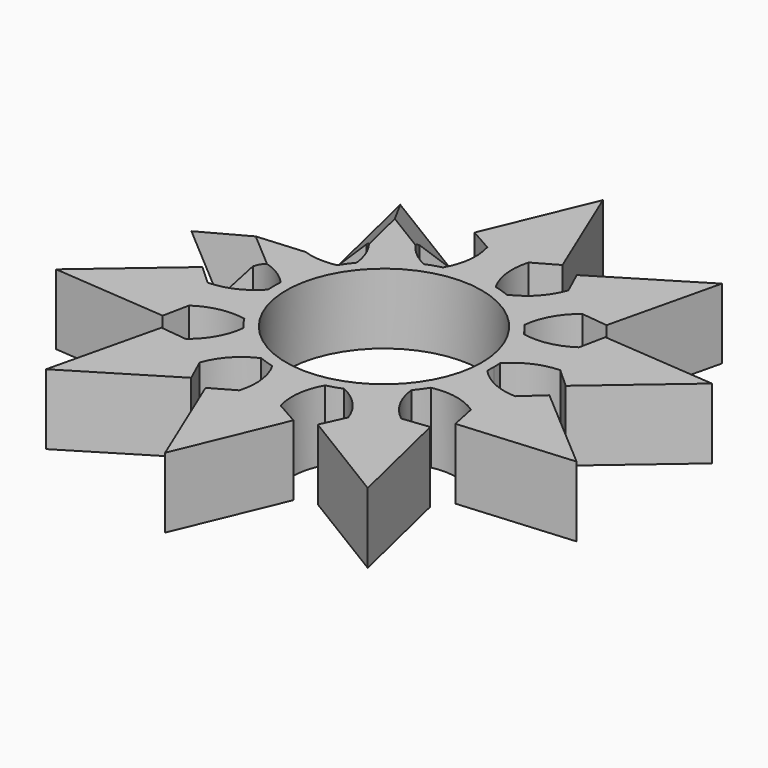
from build123d import *

# Parameters (mm, degrees)
F0_R     = 11.125
F1_DEPTH = 8
F2_SIZE  = 3.99999


# Not quite as in the source:
# - a fillet or chamfer is up to 0.001 mm smaller than in the source, because OpenCascade refuses the exact size


with BuildPart() as f1:
    # F0 (on Top) → F1 (new body)
    with BuildSketch(Plane.XY):
        with BuildLine():
            ThreePointArc((12.4677994948, -0.8966469518), (12.4919472799, -0.44861248), (12.5, 0))
            ThreePointArc((12.5, 0), (12.4919472799, 0.44861248), (12.4677994948, 0.8966469518))
            ThreePointArc((12.4677994948, 0.8966469518), (11.8882064537, 3.8627124297), (10.6136975286, 6.6029860496))
            ThreePointArc((10.6136975286, 6.6029860496), (10.1127124297, 7.3473156537), (9.559625819, 8.0537912936))
            ThreePointArc((9.559625819, 8.0537912936), (7.3473156537, 10.1127124297), (4.7055238527, 11.5805028074))
            ThreePointArc((4.7055238527, 11.5805028074), (3.8627124297, 11.8882064537), (3, 12.1346610995))
            ThreePointArc((3, 12.1346610995), (0, 12.5), (-3, 12.1346610995))
            ThreePointArc((-3, 12.1346610995), (-3.8627124297, 11.8882064537), (-4.7055238527, 11.5805028074))
            ThreePointArc((-4.7055238527, 11.5805028074), (-7.3473156537, 10.1127124297), (-9.559625819, 8.0537912936))
            ThreePointArc((-9.559625819, 8.0537912936), (-10.1127124297, 7.3473156537), (-10.6136975286, 6.6029860496))
            ThreePointArc((-10.6136975286, 6.6029860496), (-11.8882064537, 3.8627124297), (-12.4677994948, 0.8966469518))
            ThreePointArc((-12.4677994948, 0.8966469518), (-12.5, 0), (-12.4677994948, -0.8966469518))
            ThreePointArc((-12.4677994948, -0.8966469518), (-11.8882064537, -3.8627124297), (-10.6136975286, -6.6029860496))
            ThreePointArc((-10.6136975286, -6.6029860496), (-10.1127124297, -7.3473156537), (-9.559625819, -8.0537912936))
            ThreePointArc((-9.559625819, -8.0537912936), (-7.3473156537, -10.1127124297), (-4.7055238527, -11.5805028074))
            ThreePointArc((-4.7055238527, -11.5805028074), (-3.8627124297, -11.8882064537), (-3, -12.1346610995))
            ThreePointArc((-3, -12.1346610995), (0, -12.5), (3, -12.1346610995))
            ThreePointArc((3, -12.1346610995), (3.8627124297, -11.8882064537), (4.7055238527, -11.5805028074))
            ThreePointArc((4.7055238527, -11.5805028074), (7.3473156537, -10.1127124297), (9.559625819, -8.0537912936))
            ThreePointArc((9.559625819, -8.0537912936), (10.1127124297, -7.3473156537), (10.6136975286, -6.6029860496))
            ThreePointArc((10.6136975286, -6.6029860496), (11.8882064537, -3.8627124297), (12.4677994948, -0.8966469518))
        make_face()
        Circle(F0_R, mode=Mode.SUBTRACT)
        with BuildLine():
            ThreePointArc((10.6136975286, 6.6029860496), (11.8882064537, 3.8627124297), (12.4677994948, 0.8966469518))
            ThreePointArc((12.4677994948, 0.8966469518), (14.7448297559, 2.5723295046), (17.4989772889, 3.2106477587))
            ThreePointArc((17.4989772889, 3.2106477587), (18.3165016402, 3.1827968502), (19.1251951089, 3.0597659125))
            Line((19.1251951089, 3.0597659125), (17.2710931427, 8.7661050102))
            ThreePointArc((17.2710931427, 8.7661050102), (16.689162154, 8.1912327962), (16.0441414138, 7.6881721809))
            ThreePointArc((16.0441414138, 7.6881721809), (13.4407951985, 6.5857351937), (10.6136975286, 6.6029860496))
        make_face()
        with BuildLine():
            ThreePointArc((17.4989772889, -3.2106477587), (14.7448297559, -2.5723295046), (12.4677994948, -0.8966469518))
            ThreePointArc((12.4677994948, -0.8966469518), (11.8882064537, -3.8627124297), (10.6136975286, -6.6029860496))
            ThreePointArc((10.6136975286, -6.6029860496), (13.4407951985, -6.5857351937), (16.0441414138, -7.6881721809))
            ThreePointArc((16.0441414138, -7.6881721809), (16.689162154, -8.1912327962), (17.2710931427, -8.7661050102))
            Line((17.2710931427, -8.7661050102), (19.1251951089, -3.0597659125))
            ThreePointArc((19.1251951089, -3.0597659125), (18.3165016402, -3.1827968502), (17.4989772889, -3.2106477587))
        make_face()
        with BuildLine():
            ThreePointArc((19.1251951089, 3.0597659125), (18.3165016402, 3.1827968502), (17.4989772889, 3.2106477587))
            Line((17.4989772889, 3.2106477587), (19.7432290977, 1.1576528799))
            Line((19.7432290977, 1.1576528799), (19.1251951089, 3.0597659125))
        make_face()
        with BuildLine():
            Line((19.7432290977, -1.1576528799), (17.4989772889, -3.2106477587))
            ThreePointArc((17.4989772889, -3.2106477587), (18.3165016402, -3.1827968502), (19.1251951089, -3.0597659125))
            Line((19.1251951089, -3.0597659125), (19.7432290977, -1.1576528799))
        make_face()
        with BuildLine():
            ThreePointArc((4.7055238527, 11.5805028074), (7.3473156537, 10.1127124297), (9.559625819, 8.0537912936))
            ThreePointArc((9.559625819, 8.0537912936), (10.4168405049, 10.7478517624), (12.269798608, 12.8831093804))
            ThreePointArc((12.269798608, 12.8831093804), (12.9475600548, 13.3411062792), (13.674122585, 13.7169102542))
            Line((13.674122585, 13.7169102542), (8.8200206188, 17.243621768))
            ThreePointArc((8.8200206188, 17.243621768), (8.6871299688, 16.4364899243), (8.4609888389, 15.6503716587))
            ThreePointArc((8.4609888389, 15.6503716587), (7.0028337111, 13.228272889), (4.7055238527, 11.5805028074))
        make_face()
        with BuildLine():
            Line((16.6530591539, 10.6682180428), (16.0441414138, 7.6881721809))
            ThreePointArc((16.0441414138, 7.6881721809), (16.689162154, 8.1912327962), (17.2710931427, 8.7661050102))
            Line((17.2710931427, 8.7661050102), (16.6530591539, 10.6682180428))
        make_face()
        Polygon((17.2710931427, 8.7661050102), (19.1251951089, 3.0597659125), (19.7432290977, 1.1576528799), (29.6108223213, 9.6211393939), (16.6530591539, 10.6682180428), align=None)
        with BuildLine():
            ThreePointArc((12.269798608, -12.8831093804), (10.4168405049, -10.7478517624), (9.559625819, -8.0537912936))
            ThreePointArc((9.559625819, -8.0537912936), (7.3473156537, -10.1127124297), (4.7055238527, -11.5805028074))
            ThreePointArc((4.7055238527, -11.5805028074), (7.0028337111, -13.228272889), (8.4609888389, -15.6503716587))
            ThreePointArc((8.4609888389, -15.6503716587), (8.6871299688, -16.4364899243), (8.8200206188, -17.243621768))
            Line((8.8200206188, -17.243621768), (13.674122585, -13.7169102542))
            ThreePointArc((13.674122585, -13.7169102542), (12.9475600548, -13.3411062792), (12.269798608, -12.8831093804))
        make_face()
        with BuildLine():
            ThreePointArc((17.2710931427, -8.7661050102), (16.689162154, -8.1912327962), (16.0441414138, -7.6881721809))
            Line((16.0441414138, -7.6881721809), (16.6530591539, -10.6682180428))
            Line((16.6530591539, -10.6682180428), (17.2710931427, -8.7661050102))
        make_face()
        Polygon((19.7432290977, -1.1576528799), (19.1251951089, -3.0597659125), (17.2710931427, -8.7661050102), (16.6530591539, -10.6682180428), (29.6108223213, -9.6211393939), align=None)
        with BuildLine():
            ThreePointArc((13.674122585, 13.7169102542), (12.9475600548, 13.3411062792), (12.269798608, 12.8831093804))
            Line((12.269798608, 12.8831093804), (15.2921565738, 12.5413397496))
            Line((15.2921565738, 12.5413397496), (13.674122585, 13.7169102542))
        make_face()
        with BuildLine():
            Line((15.2921565738, -12.5413397496), (12.269798608, -12.8831093804))
            ThreePointArc((12.269798608, -12.8831093804), (12.9475600548, -13.3411062792), (13.674122585, -13.7169102542))
            Line((13.674122585, -13.7169102542), (15.2921565738, -12.5413397496))
        make_face()
        with BuildLine():
            ThreePointArc((-3, 12.1346610995), (0, 12.5), (3, 12.1346610995))
            ThreePointArc((3, 12.1346610995), (2.1099722363, 14.818059953), (2.353973894, 17.6346610995))
            ThreePointArc((2.353973894, 17.6346610995), (2.6330905999, 18.403566557), (3, 19.1346610995))
            Line((3, 19.1346610995), (-3, 19.1346610995))
            ThreePointArc((-3, 19.1346610995), (-2.6330905999, 18.403566557), (-2.353973894, 17.6346610995))
            ThreePointArc((-2.353973894, 17.6346610995), (-2.1099722363, 14.818059953), (-3, 12.1346610995))
        make_face()
        with BuildLine():
            Line((7.20198663, 18.4191922726), (8.4609888389, 15.6503716587))
            ThreePointArc((8.4609888389, 15.6503716587), (8.6871299688, 16.4364899243), (8.8200206188, 17.243621768))
            Line((8.8200206188, 17.243621768), (7.20198663, 18.4191922726))
        make_face()
        Polygon((8.8200206188, 17.243621768), (13.674122585, 13.7169102542), (15.2921565738, 12.5413397496), (18.3004946294, 25.1884699436), (7.20198663, 18.4191922726), align=None)
        with BuildLine():
            ThreePointArc((2.353973894, -17.6346610995), (2.1099722363, -14.818059953), (3, -12.1346610995))
            ThreePointArc((3, -12.1346610995), (0, -12.5), (-3, -12.1346610995))
            ThreePointArc((-3, -12.1346610995), (-2.1099722363, -14.818059953), (-2.353973894, -17.6346610995))
            ThreePointArc((-2.353973894, -17.6346610995), (-2.6330905999, -18.403566557), (-3, -19.1346610995))
            Line((-3, -19.1346610995), (3, -19.1346610995))
            ThreePointArc((3, -19.1346610995), (2.6330905999, -18.403566557), (2.353973894, -17.6346610995))
        make_face()
        with BuildLine():
            ThreePointArc((8.8200206188, -17.243621768), (8.6871299688, -16.4364899243), (8.4609888389, -15.6503716587))
            Line((8.4609888389, -15.6503716587), (7.20198663, -18.4191922726))
            Line((7.20198663, -18.4191922726), (8.8200206188, -17.243621768))
        make_face()
        Polygon((15.2921565738, -12.5413397496), (13.674122585, -13.7169102542), (8.8200206188, -17.243621768), (7.20198663, -18.4191922726), (18.3004946294, -25.1884699436), align=None)
        with BuildLine():
            ThreePointArc((3, 19.1346610995), (2.6330905999, 18.403566557), (2.353973894, 17.6346610995))
            Line((2.353973894, 17.6346610995), (5, 19.1346610995))
            Line((5, 19.1346610995), (3, 19.1346610995))
        make_face()
        with BuildLine():
            Line((5, -19.1346610995), (2.353973894, -17.6346610995))
            ThreePointArc((2.353973894, -17.6346610995), (2.6330905999, -18.403566557), (3, -19.1346610995))
            Line((3, -19.1346610995), (5, -19.1346610995))
        make_face()
        with BuildLine():
            ThreePointArc((-9.559625819, 8.0537912936), (-7.3473156537, 10.1127124297), (-4.7055238527, 11.5805028074))
            ThreePointArc((-4.7055238527, 11.5805028074), (-7.0028337111, 13.228272889), (-8.4609888389, 15.6503716587))
            ThreePointArc((-8.4609888389, 15.6503716587), (-8.6871299688, 16.4364899243), (-8.8200206188, 17.243621768))
            Line((-8.8200206188, 17.243621768), (-13.674122585, 13.7169102542))
            ThreePointArc((-13.674122585, 13.7169102542), (-12.9475600548, 13.3411062792), (-12.269798608, 12.8831093804))
            ThreePointArc((-12.269798608, 12.8831093804), (-10.4168405049, 10.7478517624), (-9.559625819, 8.0537912936))
        make_face()
        with BuildLine():
            Line((-5, 19.1346610995), (-2.353973894, 17.6346610995))
            ThreePointArc((-2.353973894, 17.6346610995), (-2.6330905999, 18.403566557), (-3, 19.1346610995))
            Line((-3, 19.1346610995), (-5, 19.1346610995))
        make_face()
        Polygon((-3, 19.1346610995), (3, 19.1346610995), (5, 19.1346610995), (0, 31.1346610995), (-5, 19.1346610995), align=None)
        with BuildLine():
            ThreePointArc((-8.4609888389, -15.6503716587), (-7.0028337111, -13.228272889), (-4.7055238527, -11.5805028074))
            ThreePointArc((-4.7055238527, -11.5805028074), (-7.3473156537, -10.1127124297), (-9.559625819, -8.0537912936))
            ThreePointArc((-9.559625819, -8.0537912936), (-10.4168405049, -10.7478517624), (-12.269798608, -12.8831093804))
            ThreePointArc((-12.269798608, -12.8831093804), (-12.9475600548, -13.3411062792), (-13.674122585, -13.7169102542))
            Line((-13.674122585, -13.7169102542), (-8.8200206188, -17.243621768))
            ThreePointArc((-8.8200206188, -17.243621768), (-8.6871299688, -16.4364899243), (-8.4609888389, -15.6503716587))
        make_face()
        with BuildLine():
            ThreePointArc((-3, -19.1346610995), (-2.6330905999, -18.403566557), (-2.353973894, -17.6346610995))
            Line((-2.353973894, -17.6346610995), (-5, -19.1346610995))
            Line((-5, -19.1346610995), (-3, -19.1346610995))
        make_face()
        Polygon((5, -19.1346610995), (3, -19.1346610995), (-3, -19.1346610995), (-5, -19.1346610995), (0, -31.1346610995), align=None)
        with BuildLine():
            ThreePointArc((-8.8200206188, 17.243621768), (-8.6871299688, 16.4364899243), (-8.4609888389, 15.6503716587))
            Line((-8.4609888389, 15.6503716587), (-7.20198663, 18.4191922726))
            Line((-7.20198663, 18.4191922726), (-8.8200206188, 17.243621768))
        make_face()
        with BuildLine():
            Line((-7.20198663, -18.4191922726), (-8.4609888389, -15.6503716587))
            ThreePointArc((-8.4609888389, -15.6503716587), (-8.6871299688, -16.4364899243), (-8.8200206188, -17.243621768))
            Line((-8.8200206188, -17.243621768), (-7.20198663, -18.4191922726))
        make_face()
        with BuildLine():
            ThreePointArc((-12.4677994948, 0.8966469518), (-11.8882064537, 3.8627124297), (-10.6136975286, 6.6029860496))
            ThreePointArc((-10.6136975286, 6.6029860496), (-13.4407951985, 6.5857351937), (-16.0441414138, 7.6881721809))
            ThreePointArc((-16.0441414138, 7.6881721809), (-16.689162154, 8.1912327962), (-17.2710931427, 8.7661050102))
            Line((-17.2710931427, 8.7661050102), (-19.1251951089, 3.0597659125))
            ThreePointArc((-19.1251951089, 3.0597659125), (-18.3165016402, 3.1827968502), (-17.4989772889, 3.2106477587))
            ThreePointArc((-17.4989772889, 3.2106477587), (-14.7448297559, 2.5723295046), (-12.4677994948, 0.8966469518))
        make_face()
        with BuildLine():
            Line((-15.2921565738, 12.5413397496), (-12.269798608, 12.8831093804))
            ThreePointArc((-12.269798608, 12.8831093804), (-12.9475600548, 13.3411062792), (-13.674122585, 13.7169102542))
            Line((-13.674122585, 13.7169102542), (-15.2921565738, 12.5413397496))
        make_face()
        Polygon((-13.674122585, 13.7169102542), (-8.8200206188, 17.243621768), (-7.20198663, 18.4191922726), (-18.3004946294, 25.1884699436), (-15.2921565738, 12.5413397496), align=None)
        with BuildLine():
            ThreePointArc((-16.0441414138, -7.6881721809), (-13.4407951985, -6.5857351937), (-10.6136975286, -6.6029860496))
            ThreePointArc((-10.6136975286, -6.6029860496), (-11.8882064537, -3.8627124297), (-12.4677994948, -0.8966469518))
            ThreePointArc((-12.4677994948, -0.8966469518), (-14.7448297559, -2.5723295046), (-17.4989772889, -3.2106477587))
            ThreePointArc((-17.4989772889, -3.2106477587), (-18.3165016402, -3.1827968502), (-19.1251951089, -3.0597659125))
            Line((-19.1251951089, -3.0597659125), (-17.2710931427, -8.7661050102))
            ThreePointArc((-17.2710931427, -8.7661050102), (-16.689162154, -8.1912327962), (-16.0441414138, -7.6881721809))
        make_face()
        with BuildLine():
            ThreePointArc((-13.674122585, -13.7169102542), (-12.9475600548, -13.3411062792), (-12.269798608, -12.8831093804))
            Line((-12.269798608, -12.8831093804), (-15.2921565738, -12.5413397496))
            Line((-15.2921565738, -12.5413397496), (-13.674122585, -13.7169102542))
        make_face()
        Polygon((-7.20198663, -18.4191922726), (-8.8200206188, -17.243621768), (-13.674122585, -13.7169102542), (-15.2921565738, -12.5413397496), (-18.3004946294, -25.1884699436), align=None)
        with BuildLine():
            ThreePointArc((-17.2710931427, 8.7661050102), (-16.689162154, 8.1912327962), (-16.0441414138, 7.6881721809))
            Line((-16.0441414138, 7.6881721809), (-16.6530591539, 10.6682180428))
            Line((-16.6530591539, 10.6682180428), (-17.2710931427, 8.7661050102))
        make_face()
        with BuildLine():
            Line((-16.6530591539, -10.6682180428), (-16.0441414138, -7.6881721809))
            ThreePointArc((-16.0441414138, -7.6881721809), (-16.689162154, -8.1912327962), (-17.2710931427, -8.7661050102))
            Line((-17.2710931427, -8.7661050102), (-16.6530591539, -10.6682180428))
        make_face()
        with BuildLine():
            Line((-19.7432290977, 1.1576528799), (-17.4989772889, 3.2106477587))
            ThreePointArc((-17.4989772889, 3.2106477587), (-18.3165016402, 3.1827968502), (-19.1251951089, 3.0597659125))
            Line((-19.1251951089, 3.0597659125), (-19.7432290977, 1.1576528799))
        make_face()
        Polygon((-19.1251951089, 3.0597659125), (-17.2710931427, 8.7661050102), (-16.6530591539, 10.6682180428), (-29.6108223213, 9.6211393939), (-19.7432290977, 1.1576528799), align=None)
        with BuildLine():
            ThreePointArc((-19.1251951089, -3.0597659125), (-18.3165016402, -3.1827968502), (-17.4989772889, -3.2106477587))
            Line((-17.4989772889, -3.2106477587), (-19.7432290977, -1.1576528799))
            Line((-19.7432290977, -1.1576528799), (-19.1251951089, -3.0597659125))
        make_face()
        Polygon((-16.6530591539, -10.6682180428), (-17.2710931427, -8.7661050102), (-19.1251951089, -3.0597659125), (-19.7432290977, -1.1576528799), (-29.6108223213, -9.6211393939), align=None)
    extrude(amount=F1_DEPTH)

    # F2 (size 4 in the source; OpenCascade refuses exactly that, so slightly less here)
    f2_edges = [f1.edges().sort_by_distance(p)[0] for p in [
        (-16.796326, 18.864905, 8),
        (-12.751241, 21.803831, 8),
        (-12.751241, 21.803831, 0),
        (-16.796326, 18.864905, 0),
        (-23.131941, 10.144679, 8),
        (-24.677026, 5.389396, 8),
        (-24.677026, 5.389396, 0),
        (-23.131941, 10.144679, 0),
    ]]
    chamfer(f2_edges, length=F2_SIZE)


solid = f1.part
